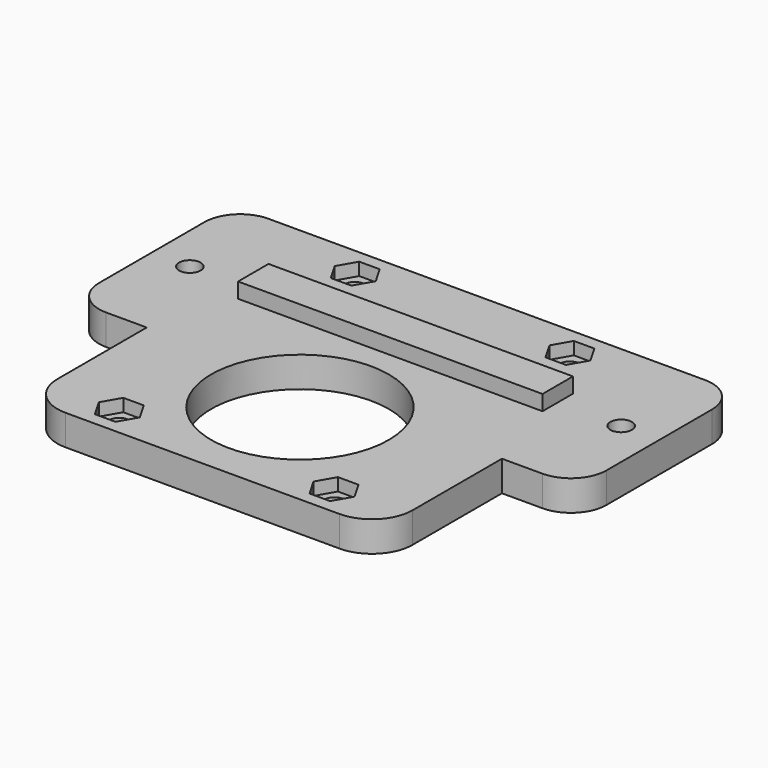
from build123d import *

# Parameters (mm, degrees)
F0_R      = 2.05
F1_DEPTH  = 6
F2_R      = 2.125
F2_W      = 60
F2_H      = 7.5
F3_DEPTH  = 6
F5_DEPTH  = 2.5
F6_DEPTH  = 25
F7_SIZE   = 1.9
F8_DEPTH  = 3
F9_R      = 17.5
F10_DEPTH = 25


# Not quite as in the source:
# - a feature names something its author has since deleted; it is built from what else it names


with BuildPart() as f1:
    # F0 (on Top) → F1 (new body)
    with BuildSketch(Plane.XY):
        with BuildLine():
            ThreePointArc((35, 27), (32.6568542495, 32.6568542495), (27, 35))
            Line((27, 35), (-27, 35))
            ThreePointArc((-27, 35), (-32.6568542495, 32.6568542495), (-35, 27))
            Line((-35, 27), (-35, -27))
            ThreePointArc((-35, -27), (-32.6568542495, -32.6568542495), (-27, -35))
            Line((-27, -35), (27, -35))
            ThreePointArc((27, -35), (32.6568542495, -32.6568542495), (35, -27))
            Line((35, -27), (35, 27))
        make_face()
        with Locations((-21.2, -29)):
            Circle(F0_R, mode=Mode.SUBTRACT)
        with Locations((21.2, -29)):
            Circle(F0_R, mode=Mode.SUBTRACT)
        with Locations((-21.2, 29)):
            Circle(F0_R, mode=Mode.SUBTRACT)
        with Locations((21.2, 29)):
            Circle(F0_R, mode=Mode.SUBTRACT)
        with Locations((-21.2, 29)):
            Circle(F0_R)
        with Locations((21.2, 29)):
            Circle(F0_R)
        with Locations((21.2, -29)):
            Circle(F0_R)
        with Locations((-21.2, -29)):
            Circle(F0_R)
    extrude(amount=-F1_DEPTH)

    # F2 (on Top) → F3 (join)
    with BuildSketch(Plane.XY):
        with BuildLine():
            ThreePointArc((50, 28), (47.9497474683, 32.9497474683), (43, 35))
            Line((43, 35), (-43, 35))
            ThreePointArc((-43, 35), (-47.9497474683, 32.9497474683), (-50, 28))
            Line((-50, 28), (-50, 2))
            ThreePointArc((-50, 2), (-47.9497474683, -2.9497474683), (-43, -5))
            Line((-43, -5), (43, -5))
            ThreePointArc((43, -5), (47.9497474683, -2.9497474683), (50, 2))
            Line((50, 2), (50, 28))
        make_face()
        with Locations((-42.5, 15)):
            Circle(F2_R, mode=Mode.SUBTRACT)
        with Locations((0, 15)):
            Rectangle(F2_W, F2_H, mode=Mode.SUBTRACT)
        with Locations((42.5, 15)):
            Circle(F2_R, mode=Mode.SUBTRACT)
    extrude(amount=-F3_DEPTH)

    # F4 (on Top) → F5 (cut)
    with BuildSketch(Plane.XY):
        Polygon((19.1289578016, -32.5574766695), (23.1704096859, -32.5574766695), (25.191135628, -29.0574766695), (23.1704096859, -25.5574766695), (19.1289578016, -25.5574766695), (17.1082318594, -29.0574766695), align=None)
        Polygon((-17.1082318594, -29.0574766695), (-19.1289578016, -25.5574766695), (-23.1704096859, -25.5574766695), (-25.191135628, -29.0574766695), (-23.1704096859, -32.5574766695), (-19.1289578016, -32.5574766695), align=None)
        Polygon((-23.1704096859, 25.5574766695), (-19.1289578016, 25.5574766695), (-17.1082318594, 29.0574766695), (-19.1289578016, 32.5574766695), (-23.1704096859, 32.5574766695), (-25.191135628, 29.0574766695), align=None)
        Polygon((19.1289578016, 32.5574766695), (17.1082318594, 29.0574766695), (19.1289578016, 25.5574766695), (23.1704096859, 25.5574766695), (25.191135628, 29.0574766695), (23.1704096859, 32.5574766695), align=None)
    extrude(amount=-F5_DEPTH, mode=Mode.SUBTRACT)

    # F0 (on Top) → F6 (cut)
    with BuildSketch(Plane.XY):
        with Locations((-21.2, 29)):
            Circle(F0_R)
        with Locations((21.2, 29)):
            Circle(F0_R)
        with Locations((21.2, -29)):
            Circle(F0_R)
        with Locations((-21.2, -29)):
            Circle(F0_R)
    extrude(amount=-F6_DEPTH, mode=Mode.SUBTRACT)

    # F7
    f7_edges = [f1.edges().sort_by_distance(p)[0] for p in [
        (40.375, 15, -6),
        (-44.625, 15, -6),
    ]]
    chamfer(f7_edges, length=F7_SIZE)

    # F2 (on Top) → F8 (join)
    with BuildSketch(Plane.XY):
        with Locations((0, 15)):
            Rectangle(F2_W, F2_H)
    extrude(amount=F8_DEPTH)

    # F9 (on Top) → F10 (cut)
    with BuildSketch(Plane.XY):
        with Locations((0, -11)):
            Circle(F9_R)
    extrude(amount=-F10_DEPTH, mode=Mode.SUBTRACT)


solid = f1.part
